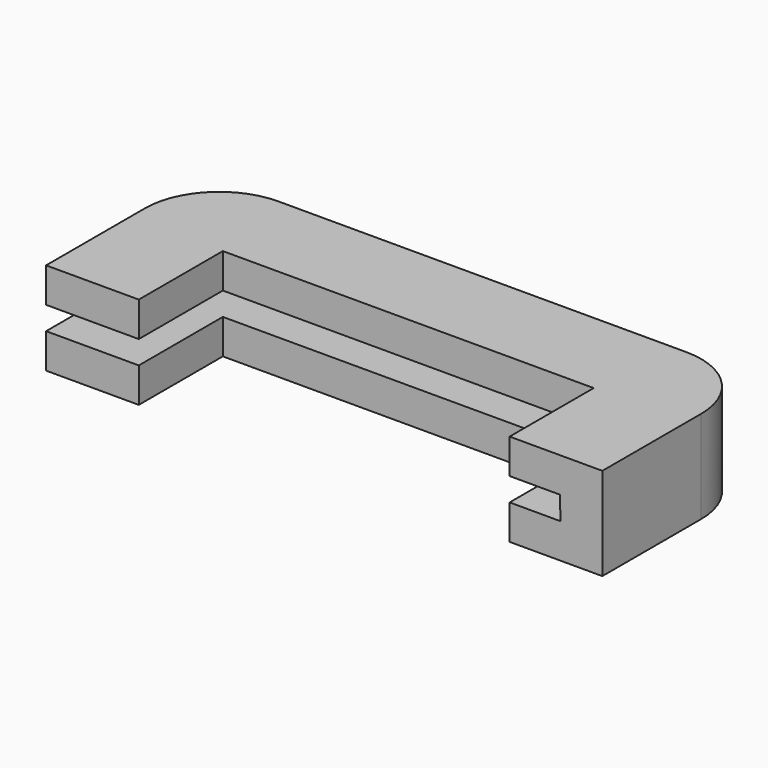
from build123d import *

# Parameters (mm, degrees)
F0_W        = 6.35
F0_H        = 6.35
F0_H_2      = 7.196190767
F1_DEPTH    = 6.35
F2_W        = 6.35
F2_H        = 1.5875
F3_DEPTH    = 9.779
F4_T1_DEPTH = 31.75


# Not quite as in the source:
# - a fillet or chamfer that OpenCascade refuses, or shapes differently, is made with other operations: its cross-section is extruded or revolved along the edge and cut away or added


with BuildPart() as f1:
    # F0 (on Top) → F1 (new body)
    with BuildSketch(Plane.XY):
        Polygon((-12.7, 13.546190767), (-12.7, 7.196190767), (0, 7.196190767), (12.7, 7.196190767), (12.7, 13.546190767), align=None)
        with Locations((-15.875, 10.371190767)):
            Rectangle(F0_W, F0_H)
        with Locations((-15.875, 3.5980953835)):
            Rectangle(F0_W, F0_H_2)
        with Locations((15.875, 10.371190767)):
            Rectangle(F0_W, F0_H)
        with Locations((15.875, 3.5980953835)):
            Rectangle(F0_W, F0_H_2)
    extrude(amount=F1_DEPTH)

    # F2 (on face) → F3 (cut)
    with BuildSketch(Plane.XZ):
        Polygon((9.525, 3.96875), (-8.7374933064, 3.96875), (-12.7, 3.96875), (-12.7, 2.38125), (-8.7374933064, 2.38125), (9.525, 2.38125), align=None)
        Polygon((16.1540079862, 3.96875), (9.525, 3.96875), (9.525, 2.38125), (16.1763634533, 2.38125), align=None)
        with Locations((-15.875, 3.175)):
            Rectangle(F2_W, F2_H)
    extrude(amount=-F3_DEPTH, mode=Mode.SUBTRACT)

    # F4: fillet of radius 5.08 on 2 edges, made by hand

    # F4_s2 → F4_t1 (cut)
    with BuildSketch(Plane.XY.offset(-12.7)):
        with BuildLine():
            ThreePointArc((13.97, 13.546190767), (17.5621024484, 12.0582932154), (19.05, 8.466190767))
            Line((19.05, 8.466190767), (19.05, 13.546190767))
            Line((19.05, 13.546190767), (13.97, 13.546190767))
        make_face()
        with BuildLine():
            ThreePointArc((-19.05, 8.466190767), (-17.5621024484, 12.0582932154), (-13.97, 13.546190767))
            Line((-13.97, 13.546190767), (-19.05, 13.546190767))
            Line((-19.05, 13.546190767), (-19.05, 8.466190767))
        make_face()
    extrude(amount=F4_T1_DEPTH, mode=Mode.SUBTRACT)


solid = f1.part
